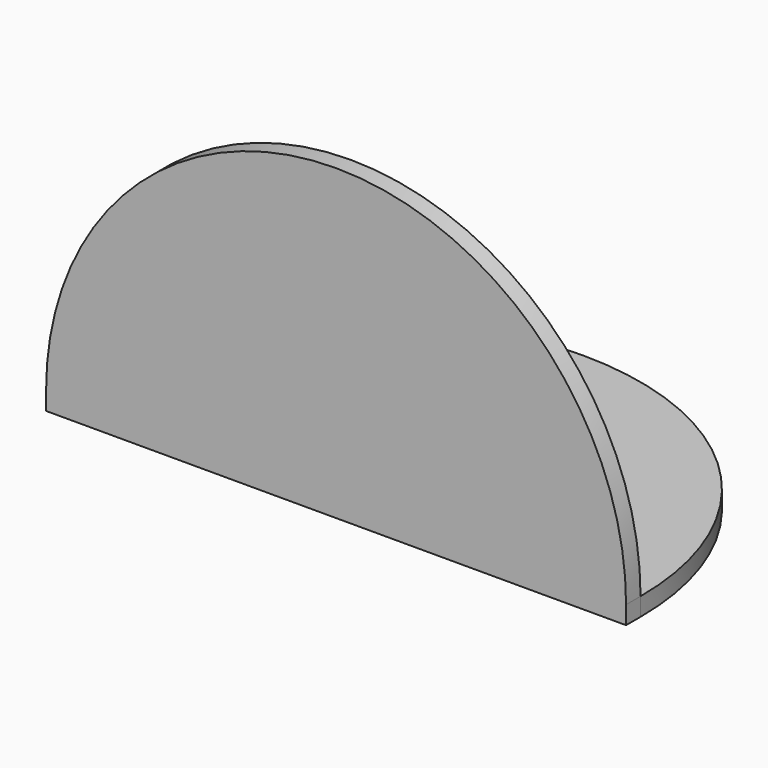
from build123d import *

# Parameters (mm, degrees)
F1_DEPTH      = 3.175
F3_DEPTH      = 3.175
F4_W          = 3.175
F4_H          = 3.175
F5_DEPTH      = 50.8
F5_DEPTH_BACK = 50.8


# Not quite as in the source:
# - an extrude ends at something that could not be found from the text; its depth is read off the source's solid


with BuildPart() as f1:
    # F0 (on Top) → F1 (new body)
    with BuildSketch(Plane.XY):
        with BuildLine():
            Line((-50.8, 0), (50.8, 0))
            ThreePointArc((50.8, 0), (0, 50.8), (-50.8, 0))
        make_face()
    extrude(amount=F1_DEPTH)

    # F2 (on face) → F3 (join)
    with BuildSketch(Plane.XZ):
        with BuildLine():
            ThreePointArc((50.8, 3.175), (0, 53.975), (-50.8, 3.175))
            Line((-50.8, 3.175), (50.8, 3.175))
        make_face()
    extrude(amount=F3_DEPTH)

    # F4 (on Right) → F5 (join, two sides)
    with BuildSketch(Plane.YZ) as f5_sk:
        with Locations((-1.5875, 1.5875)):
            Rectangle(F4_W, F4_H)
    extrude(amount=F5_DEPTH)
    extrude(f5_sk.sketch, amount=-F5_DEPTH_BACK)


solid = f1.part
